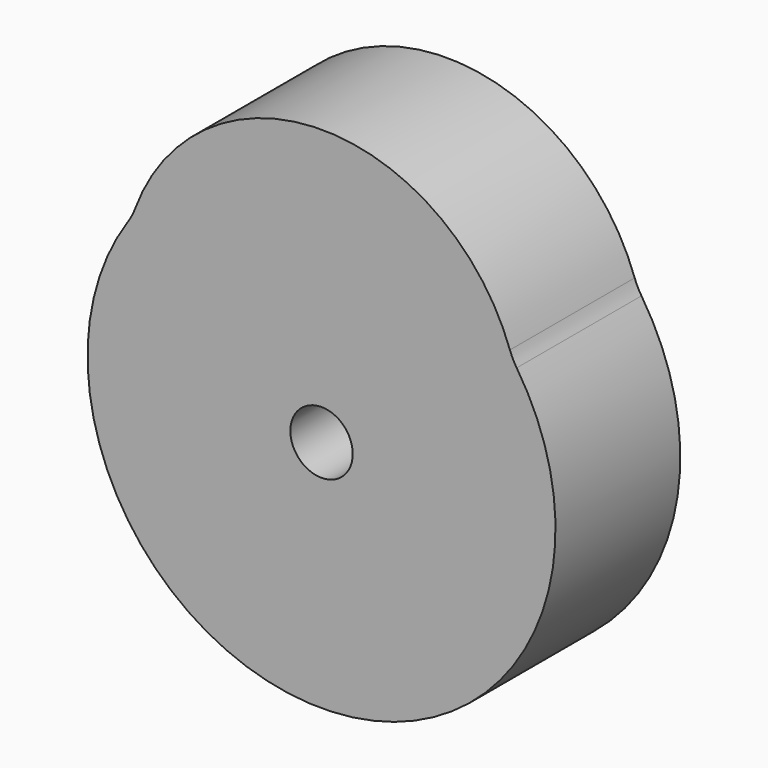
from build123d import *

# Parameters (mm, degrees)
F1_DEPTH = 12.5
F2_R     = 10
F3_R     = 5
F4_DEPTH = 25.0010001


with BuildPart() as f1:
    # F0 (on Front) → F1 (new body, symmetric)
    with BuildSketch(Plane.XZ):
        with BuildLine():
            ThreePointArc((30.5734569437, 21.7143669149), (0.2987295857, 44.1480604907), (-30.2768086166, 22.1261126273))
            ThreePointArc((-30.2768086166, 22.1261126273), (-0.2537394144, -37.499141541), (30.5734569437, 21.7143669149))
        make_face()
    extrude(amount=F1_DEPTH, both=True)

    # F2
    f2_edges = [f1.edges().sort_by_distance(p)[0] for p in [
        (-30.276809, 0, 22.126113),
        (30.573457, 0, 21.714367),
    ]]
    fillet(f2_edges, radius=F2_R)

    # F3 (on face) → F4 (cut, through all)
    with BuildSketch(Plane.XZ.offset(12.5)):
        Circle(F3_R)
    extrude(amount=-F4_DEPTH, mode=Mode.SUBTRACT)


solid = f1.part
